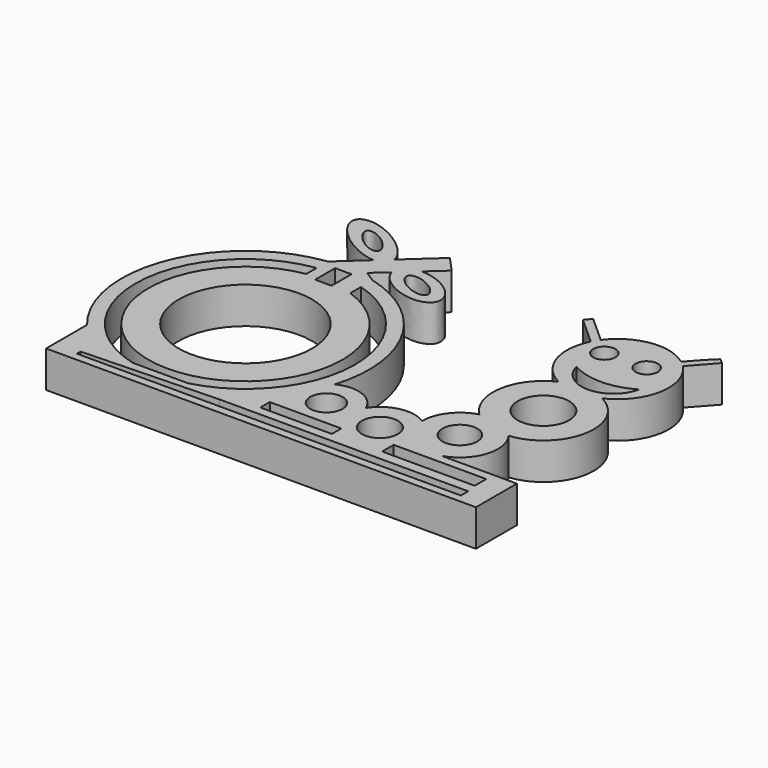
from build123d import *

# Parameters (mm, degrees)
F0_R     = 46.2337285332
F0_W     = 49.6600195765
F0_H     = 8.200738579
F0_R_2   = 11.2330932007
F0_R_3   = 12.5096021804
F0_W_2   = 64.2391070724
F0_H_2   = 10.0231207907
F0_R_4   = 12.1110753235
F0_R_5   = 17.8847335495
F0_W_3   = 11.3898105919
F0_H_3   = 17.3125043511
F0_R_6   = 7.7451318502
F0_R_7   = 7.7852341734
F1_DEPTH = 25.4


# Not quite as in the source:
# - a feature names something its author has since deleted; it is built from what else it names


with BuildPart() as f1:
    # F0 (on Top) → F1 (new body)
    with BuildSketch(Plane.XY):
        with BuildLine():
            ThreePointArc((107.7295786753, -13.8945599229), (89.6079290098, -10.5687529062), (74.4358429591, -21.0216464664))
            ThreePointArc((74.4358429591, -21.0216464664), (61.6395998633, -8.9177051648), (44.054970235, -9.9326106946))
            ThreePointArc((44.054970235, -9.9326106946), (44.0216607871, -9.94936839), (43.9883795128, -9.9661819695))
            ThreePointArc((43.9883795128, -9.9661819695), (36.8725672934, 56.9733368671), (-16.332254, 98.2138625276))
            Line((-16.332254, 98.2138625276), (-16.4762551684, 98.307190481))
            Line((-16.4762551684, 98.307190481), (-24.0230032828, 103.1982796597))
            Line((-24.0230032828, 103.1982796597), (-14.1585315489, 112.0846304755))
            add(Edge.make_bspline(
                [(-14.1585315489, 112.0846304755), (-3.5576970286, 72.2876572961), (24.625568708, 97.676384967), (52.8088344446, 123.0651126378), (-2.0455294039, 122.9965565671)],
                knots=[0.4101280656, 0.4101280656, 0.4101280656, 2.8837866972, 2.8837866972, 5.3574453288, 5.3574453288, 5.3574453288], degree=2, weights=[1, 0.3277934292, 1, 0.3277934292, 1]))
            Line((-2.0455294039, 122.9965565671), (10.0420509966, 133.8855816309))
            Line((10.0420509966, 133.8855816309), (0, 144.9297015087))
            Line((0, 144.9297015087), (-22.3107314265, 124.6432952369))
            add(Edge.make_bspline(
                [(-22.3107314265, 124.6432952369), (-25.6343535574, 141.9088069841), (-52.3630960275, 150.1852915882), (-79.0918384976, 158.4617761923), (-65.6834446446, 138.0735414818), (-52.2750507915, 117.6853067713), (-30.6053039446, 117.1013162343)],
                knots=[0.3868328797, 0.3868328797, 0.3868328797, 2.1474168151, 2.1474168151, 3.9080007506, 3.9080007506, 5.6685846861, 5.6685846861, 5.6685846861], degree=2, weights=[1, 0.6369260862, 1, 0.6369260862, 1, 0.6369260862, 1]))
            Line((-30.6053039446, 117.1013162343), (-44.997071173, 104.0153608084))
            Line((-44.997071173, 104.0153608084), (-48.9817820908, 100.3921956594))
            Line((-48.9817820908, 100.3921956594), (-49.0512791846, 100.3290042627))
            ThreePointArc((-49.0512791846, 100.3290042627), (-117.9299183099, 46.8738666151), (-104.5476059195, -39.2808336848))
            Line((-104.5476059195, -39.2808336848), (-104.5476059195, -39.3657855206))
            Line((-104.5476059195, -39.3657855206), (-104.5476059195, -74.7953727841))
            Line((-104.5476059195, -74.7953727841), (193.8383877277, -74.7953727841))
            Line((193.8383877277, -74.7953727841), (193.8383877277, -39.2808336848))
            Line((193.8383877277, -39.2808336848), (141.6114676661, -39.2808336848))
            ThreePointArc((141.6114676661, -39.2808336848), (159.1188181407, -22.3156937595), (155.2330489218, 1.7513810711))
            ThreePointArc((155.2330489218, 1.7513810711), (186.0115295128, 30.2314569619), (167.3389228513, 67.7782724153))
            ThreePointArc((167.3389228513, 67.7782724153), (187.3220194013, 93.4637146547), (177.8728575709, 124.6049964436))
            Line((177.8728575709, 124.6049964436), (192.2312635884, 140.6526330346))
            Line((192.2312635884, 140.6526330346), (188.7724029248, 143.7474018801))
            Line((188.7724029248, 143.7474018801), (182.4195683002, 137.5578641892))
            Line((182.4195683002, 137.5578641892), (173.9410394456, 128.0818576101))
            ThreePointArc((173.9410394456, 128.0818576101), (147.4497947633, 134.9255089971), (123.9992773109, 120.8295932647))
            Line((123.9992773109, 120.8295932647), (105.3029671311, 137.5578641892))
            Line((105.3029671311, 137.5578641892), (101.6390184169, 133.2566856372))
            Line((101.6390184169, 133.2566856372), (120.9925508075, 115.9403740195))
            ThreePointArc((120.9925508075, 115.9403740195), (118.9482902232, 88.7875103825), (136.7977876196, 68.2241340128))
            ThreePointArc((136.7977876196, 68.2241340128), (117.1185074951, 42.3459026602), (127.2393729637, 11.4505145524))
            ThreePointArc((127.2393729637, 11.4505145524), (113.202453066, 2.0741358303), (107.7295786753, -13.8945599229))
        make_face()
        with Locations((-38.1296895495, 15.1524662187)):
            Circle(F0_R, mode=Mode.SUBTRACT)
        with BuildLine():
            Line((-16.332254, 82.0587446918), (-16.332254, 88.2035223783))
            ThreePointArc((-16.332254, 88.2035223783), (38.0917367076, 13.7816336616), (-18.9731285161, -58.635142307))
            Line((-18.9731285161, -58.635142307), (-57.2862505829, -58.635142307))
            ThreePointArc((-57.2862505829, -58.635142307), (-114.2476415826, 19.3527496442), (-49.0512791846, 90.5998245715))
            Line((-49.0512791846, 90.5998245715), (-49.0512791846, 84.6671925398))
            Line((-49.0512791846, 84.6671925398), (-49.0512791846, 81.5833761946))
            ThreePointArc((-49.0512791846, 81.5833761946), (-43.7368749443, -51.9363286157), (-16.332254, 78.8487669264))
            Line((-16.332254, 78.8487669264), (-16.332254, 82.0587446918))
        make_face(mode=Mode.SUBTRACT)
        Polygon((-87.6497253776, -65.949074924), (6.2565519474, -62.759898603), (178.8742244244, -62.759898603), (178.8742244244, -69.138251245), (-87.6497253776, -69.138251245), align=None, mode=Mode.SUBTRACT)
        with Locations((54.2685873806, -52.281184122)):
            Rectangle(F0_W, F0_H, mode=Mode.SUBTRACT)
        with Locations((54.0224537253, -29.7865662724)):
            Circle(F0_R_2, mode=Mode.SUBTRACT)
        with Locations((94.6506485343, -34.1254994273)):
            Circle(F0_R_3, mode=Mode.SUBTRACT)
        with Locations((145.38789168, -50.458798185)):
            Rectangle(F0_W_2, F0_H_2, mode=Mode.SUBTRACT)
        with Locations((134.0954899788, -14.0086282044)):
            Circle(F0_R_4, mode=Mode.SUBTRACT)
        with Locations((151.6090482473, 36.5390703082)):
            Circle(F0_R_5, mode=Mode.SUBTRACT)
        with Locations((-35.4250539094, 88.0410410464)):
            Rectangle(F0_W_3, F0_H_3, mode=Mode.SUBTRACT)
        with BuildLine():
            add(Edge.make_bspline(
                [(-35.6528498232, 126.7663836479), (-30.4327622591, 133.4271267378), (-47.5508131354, 141.4668180209), (-64.6688640118, 149.506509304), (-52.7709006996, 134.806074931), (-40.8729373874, 120.105640558), (-35.6528498232, 126.7663836479)],
                knots=[0, 0, 0, 2.0943951024, 2.0943951024, 4.1887902048, 4.1887902048, 6.2831853072, 6.2831853072, 6.2831853072], degree=2, weights=[1, 0.5, 1, 0.5, 1, 0.5, 1]))
        make_face(mode=Mode.SUBTRACT)
        with BuildLine():
            add(Edge.make_bspline(
                [(17.1958617866, 103.0755937099), (21.5584125472, 111.3794925705), (3.0210992372, 115.8203796991), (-15.5162140727, 120.2612668276), (-1.3414515233, 107.5164808385), (12.833311026, 94.7716948494), (17.1958617866, 103.0755937099)],
                knots=[0, 0, 0, 2.0943951024, 2.0943951024, 4.1887902048, 4.1887902048, 6.2831853072, 6.2831853072, 6.2831853072], degree=2, weights=[1, 0.5, 1, 0.5, 1, 0.5, 1]))
        make_face(mode=Mode.SUBTRACT)
        with BuildLine():
            ThreePointArc((176.6544133425, 88.4980857372), (155.1954693266, 70.9918250207), (133.3727687597, 88.0424901843))
            ThreePointArc((133.3727687597, 88.0424901843), (155.0747341605, 82.4616835644), (176.6544133425, 88.4980857372))
        make_face(mode=Mode.SUBTRACT)
        with Locations((135.1951658726, 109.911121428)):
            Circle(F0_R_6, mode=Mode.SUBTRACT)
        with Locations((163.8977229595, 110.8223050833)):
            Circle(F0_R_7, mode=Mode.SUBTRACT)
    extrude(amount=F1_DEPTH)


solid = f1.part
